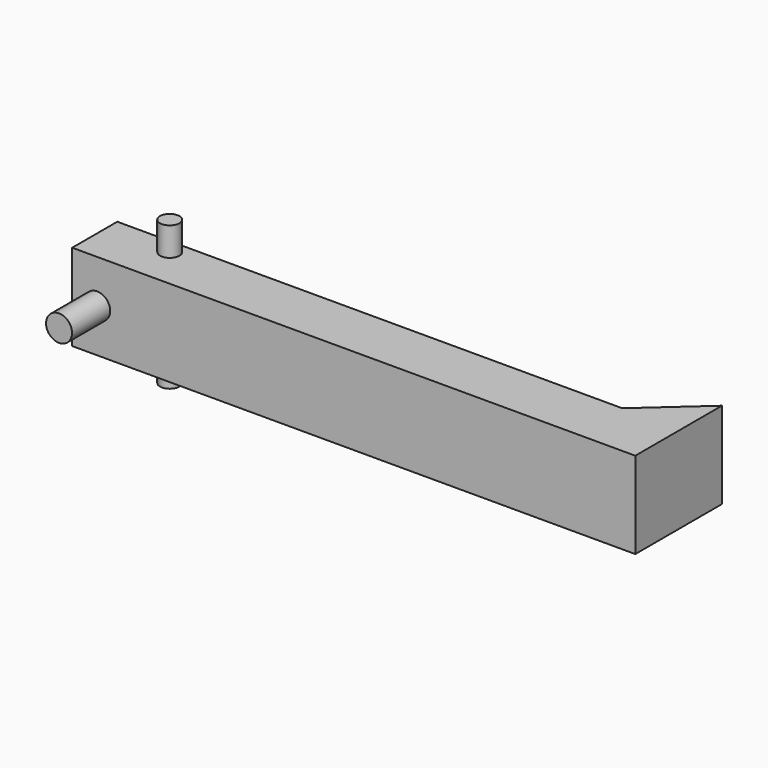
from build123d import *

# Parameters (mm, degrees)
F0_W          = 165.1
F0_H          = 25.4
F1_DEPTH      = 16.51
F2_R          = 3.81
F3_DEPTH      = 13.97
F5_R          = 2.8575
F6_DEPTH      = 8.382
F6_DEPTH_BACK = 33.782
F7_DEPTH      = 25.4


# Not quite as in the source:
# - a feature names something its author has since deleted; it is built from what else it names


with BuildPart() as f1:
    # F0 (on Front) → F1 (new body)
    with BuildSketch(Plane.XZ):
        with Locations((17.2861106694, 1.5442719363)):
            Rectangle(F0_W, F0_H)
    extrude(amount=F1_DEPTH)

    # F2 (on face) → F3 (join)
    with BuildSketch(Plane.XZ.offset(16.51)):
        with Locations((-57.9527877271, 1.5442719363)):
            Circle(F2_R)
    extrude(amount=F3_DEPTH)

    # F5 (on face) → F6 (join, two sides)
    with BuildSketch(Plane(origin=(0, 0, -11.1557280637), x_dir=(1, 0, 0), z_dir=(0, 0, -1))) as f6_sk:
        with Locations((-46.4608334005, 4.2803706601)):
            Circle(F5_R)
    extrude(amount=F6_DEPTH)
    extrude(f6_sk.sketch, amount=-F6_DEPTH_BACK)

    # F4 (on face) → F7 (join)
    with BuildSketch(Plane(origin=(0, 0, -11.1557280637), x_dir=(1, 0, 0), z_dir=(0, 0, -1))):
        Polygon((99.8361106694, 0), (82.7972726808, 0), (99.8361106694, -15.24), align=None)
    extrude(amount=-F7_DEPTH)


solid = f1.part
